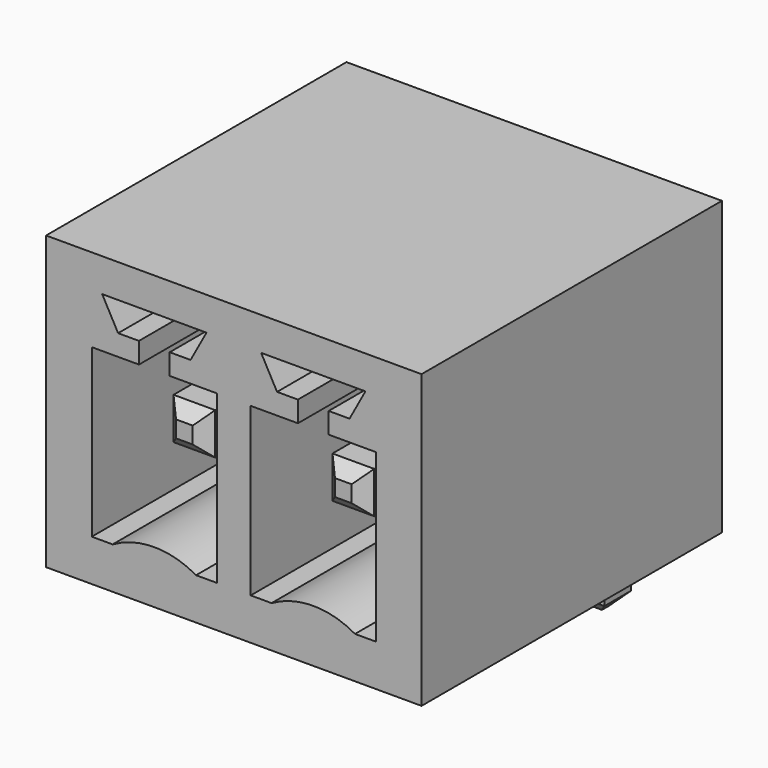
from build123d import *

# Parameters (mm, degrees)
F0_W       = 9
F0_H       = 9
F1_DEPTH   = 7
F3_DEPTH   = 8
F4_W       = 1
F4_H       = 3.8358249348
F5_DEPTH   = 0.9
F8_DEPTH   = 1
F10_DEPTH  = 1
F11_SIZE   = 0.3
F11_2_SIZE = 0.3
F13_DEPTH  = 8


# Not quite as in the source:
# - a feature names something its author has since deleted; it is built from what else it names


with BuildPart() as f1:
    # F0 (on Top) → F1 (new body)
    with BuildSketch(Plane.XY):
        Rectangle(F0_W, F0_H)
    extrude(amount=F1_DEPTH)

    # F2 (on face) → F3 (cut)
    with BuildSketch(Plane.XZ.offset(4.5)):
        Polygon((-3.405, 1), (-0.405, 1), (-0.405, 5), (-1.5365509928, 5), (-1.5365509928, 5.5), (-1.0365509928, 5.5), (-0.655, 6.2), (-3.155, 6.2), (-2.7734490072, 5.5), (-2.2734490072, 5.5), (-2.2734490072, 5), (-3.405, 5), align=None)
        Polygon((3.155, 6.2), (0.655, 6.2), (1.0365509928, 5.5), (1.5365509928, 5.5), (1.5365509928, 5), (0.405, 5), (0.405, 1), (3.405, 1), (3.405, 5), (2.2734490072, 5), (2.2734490072, 5.5), (2.7734490072, 5.5), align=None)
    extrude(amount=-F3_DEPTH, mode=Mode.SUBTRACT)

    # F4 (on face) → F5 (cut)
    with BuildSketch(Plane(origin=(0, 4.5, 0), x_dir=(-1, 0, 0), z_dir=(0, 1, 0))):
        with Locations((-1.905, 1.9179124674)):
            Rectangle(F4_W, F4_H)
        with Locations((1.905, 1.9179124674)):
            Rectangle(F4_W, F4_H)
    extrude(amount=-F5_DEPTH, mode=Mode.SUBTRACT)

    # F12 (on face) → F13 (join, through all)
    with BuildSketch(Plane.XZ.offset(4.5)):
        with BuildLine():
            Line((-2.905, 1), (-0.905, 1))
            ThreePointArc((-0.905, 1), (-1.905, 1.2679491924), (-2.905, 1))
        make_face()
        with BuildLine():
            ThreePointArc((2.905, 1), (1.905, 1.2679491924), (0.905, 1))
            Line((0.905, 1), (2.905, 1))
        make_face()
    extrude(amount=-F13_DEPTH)


with BuildPart() as f8:
    # F7 (on face) → F8 (new body)
    with BuildSketch(Plane.YZ.offset(-2.405)):
        Polygon((4.4, 3.8321887431), (-3.6, 3.8321887431), (-3.6, 2.8321887431), (3.6, 2.8321887431), (3.6, -2.1678112569), (4.4, -2.1678112569), align=None)
    extrude(amount=F8_DEPTH)

    # F11
    f11_edges = [f8.edges().sort_by_distance(p)[0] for p in [
        (-1.905, -3.6, 3.832189),
        (-1.905, -3.6, 2.832189),
        (-2.405, -3.6, 3.332189),
        (-1.405, -3.6, 3.332189),
        (-1.905, 3.6, -2.167811),
        (-1.905, 4.4, -2.167811),
        (-2.405, 4, -2.167811),
        (-1.405, 4, -2.167811),
    ]]
    chamfer(f11_edges, length=F11_SIZE)


with BuildPart() as f10:
    # F9 (on face) → F10 (new body)
    with BuildSketch(Plane.YZ.offset(1.405)):
        Polygon((3.6, -2.1678112569), (4.4, -2.1678112569), (4.4, 3.8321887431), (-3.6, 3.8321887431), (-3.6, 2.8321887431), (3.6, 2.8321887431), align=None)
    extrude(amount=F10_DEPTH)

    # F11#2
    f11_2_edges = [f10.edges().sort_by_distance(p)[0] for p in [
        (1.905, -3.6, 3.832189),
        (1.905, -3.6, 2.832189),
        (1.405, -3.6, 3.332189),
        (2.405, -3.6, 3.332189),
        (1.905, 3.6, -2.167811),
        (1.905, 4.4, -2.167811),
        (1.405, 4, -2.167811),
        (2.405, 4, -2.167811),
    ]]
    chamfer(f11_2_edges, length=F11_2_SIZE)


solid = Compound([f1.part, f8.part, f10.part])
